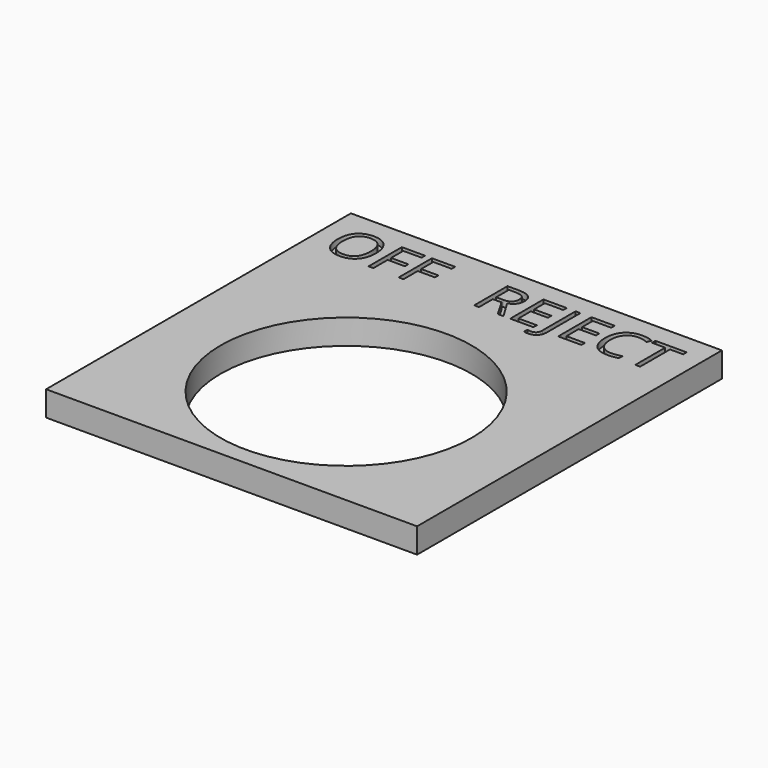
from build123d import *

# Parameters (mm, degrees)
F0_W         = 45.2628
F0_H         = 46.482
F0_R         = 15.3035
F1_DEPTH     = 3.048
F2_TEXT_SIZE = 7.1105756108
F3_DEPTH     = 0.762


# Not quite as in the source:
# - Text() gives the source's letters only with a copy of the font that has no kerning and outlines rounded to 1/6400 em; it was checked with that copy


with BuildPart() as f1:
    # F0 (on Top) → F1 (new body)
    with BuildSketch(Plane.XY):
        with Locations((0, 5.7785)):
            Rectangle(F0_W, F0_H)
        Circle(F0_R, mode=Mode.SUBTRACT)
    extrude(amount=F1_DEPTH)

    # F2 (on face) → F3 (cut)
    with BuildSketch(Plane.XY.offset(3.048)):
        with Locations((-20.7184396859, 21.529081914)):
            Text('OFF   REJECT', F2_TEXT_SIZE, font='Open Sans', text_align=(TextAlign.LEFT, TextAlign.BOTTOM))
    extrude(amount=-F3_DEPTH, mode=Mode.SUBTRACT)


solid = f1.part
